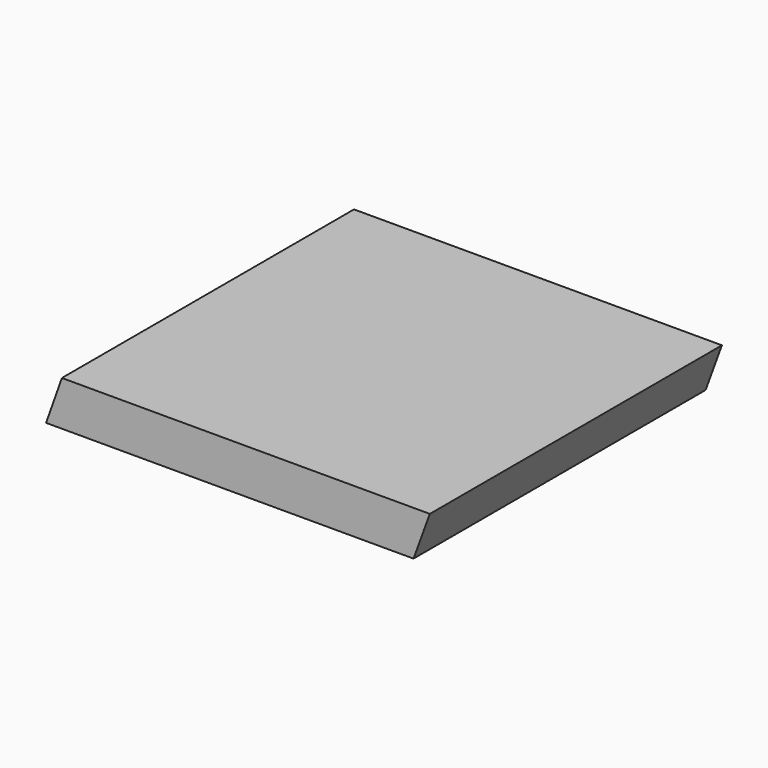
from build123d import *

# Parameters (mm, degrees)
F1_DEPTH = 2438.4


# Not quite as in the source:
# - a feature names something its author has since deleted; it is built from what else it names


with BuildPart() as f1:
    # F0 (on Front) → F1 (new body)
    with BuildSketch(Plane.XZ):
        Polygon((1244.6, 149.225), (-1063.0834102631, 149.225), (-1168.7681674957, -149.225), (1244.6, -149.225), align=None)
        Polygon((1394.166469574, 149.225), (1244.6, 149.225), (1359.1151759869, 53.1140487253), align=None)
        Polygon((1359.1151759869, 53.1140487253), (1244.6, 149.225), (1244.6, -149.225), (1285.3229045868, -149.225), align=None)
    extrude(amount=F1_DEPTH)


solid = f1.part
